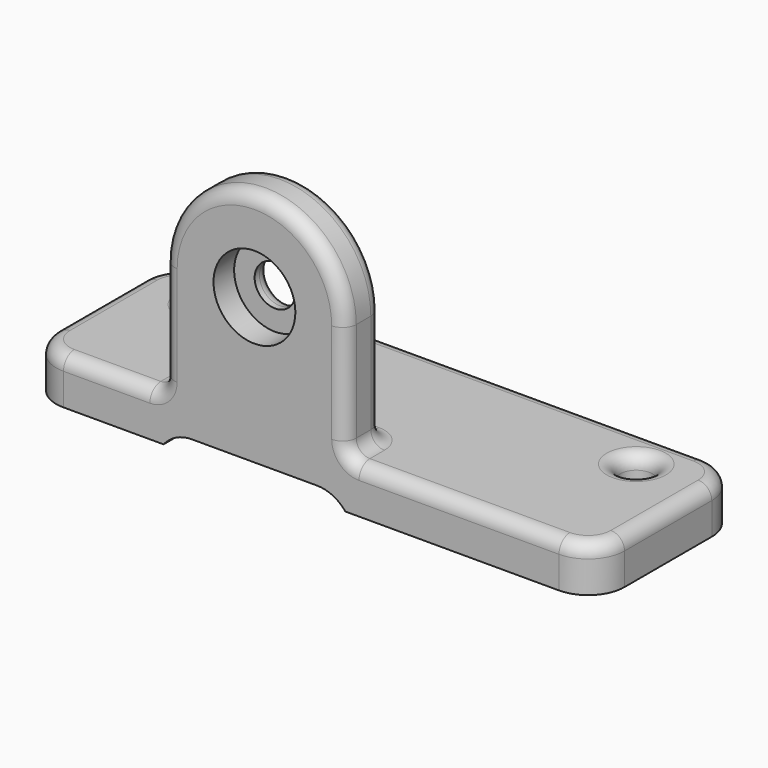
from build123d import *

# Parameters (mm, degrees)
F0_W           = 125
F0_H           = 40
F1_DEPTH       = 10
F3_DEPTH       = 10
F5_D           = 9
F5_CBORE_D     = 18.01
F5_CBORE_DEPTH = 5.68
F6_W           = 40
F6_H           = 3
F7_DEPTH       = 40.001
F8_T1_DEPTH    = 40
F9_R           = 3.2524289183
F10_DEPTH      = 10.001
F11_R          = 3.5
F12_DEPTH      = 25
F13_R          = 8
F14_R          = 3


# Not quite as in the source:
# - a fillet or chamfer that OpenCascade refuses, or shapes differently, is made with other operations: its cross-section is extruded or revolved along the edge and cut away or added


with BuildPart() as f1:
    # F0 (on Top) → F1 (new body)
    with BuildSketch(Plane.XY):
        Rectangle(F0_W, F0_H)
    extrude(amount=F1_DEPTH)

    # F2 (on face) → F3 (join)
    with BuildSketch(Plane.XZ.offset(20)):
        with BuildLine():
            Line((-32.5, 35), (-32.5, 10))
            Line((-32.5, 10), (7.5, 10))
            Line((7.5, 10), (7.5, 35))
            ThreePointArc((7.5, 35), (-12.5, 55), (-32.5, 35))
        make_face()
    extrude(amount=-F3_DEPTH)

    # F5 (through all)
    with Locations(Plane.XZ.offset(20)):
        with Locations((-12.5, 35)):
            CounterBoreHole(F5_D / 2, F5_CBORE_D / 2, F5_CBORE_DEPTH)

    # F6 (on face) → F7 (cut, through all)
    with BuildSketch(Plane.XZ.offset(20)):
        with Locations((-12.5, 1.5)):
            Rectangle(F6_W, F6_H)
    extrude(amount=-F7_DEPTH, mode=Mode.SUBTRACT)

    # F8: fillet of radius 8 on 2 edges, made by hand

    # F8_s2 → F8_t1 (join)
    with BuildSketch(Plane.XZ.offset(-20)):
        with BuildLine():
            ThreePointArc((-32.5, 0), (-29.7191036167, 2.2111025509), (-26.2550020016, 3))
            Line((-26.2550020016, 3), (-32.5, 3))
            Line((-32.5, 3), (-32.5, 0))
        make_face()
        with BuildLine():
            ThreePointArc((1.2550020016, 3), (4.7191036167, 2.2111025509), (7.5, 0))
            Line((7.5, 0), (7.5, 3))
            Line((7.5, 3), (1.2550020016, 3))
        make_face()
    extrude(amount=F8_T1_DEPTH)

    # F9 (on face) → F10 (cut, through all)
    with BuildSketch(Plane.XY.offset(10)):
        with Locations((-47.5, 10)):
            Circle(F9_R)
    extrude(amount=-F10_DEPTH, mode=Mode.SUBTRACT)

    # F11 (on face) → F12 (cut)
    with BuildSketch(Plane.XY.offset(10)):
        with Locations((47.5, 10)):
            Circle(F11_R)
    extrude(amount=-F12_DEPTH, mode=Mode.SUBTRACT)

    # F13
    f13_edges = [f1.edges().sort_by_distance(p)[0] for p in [
        (62.5, -20, 5),
        (-62.5, -20, 5),
        (-62.5, 20, 5),
        (62.5, 20, 5),
    ]]
    fillet(f13_edges, radius=F13_R)

    # F14
    f14_edges = [f1.edges().sort_by_distance(p)[0] for p in [
        (7.5, -15, 10),
        (-32.5, -15, 10),
        (-62.5, 0, 10),
        (-60.156854, 17.656854, 10),
        (-60.156854, -17.656854, 10),
        (0, 20, 10),
        (-43.5, -20, 10),
        (60.156854, 17.656854, 10),
        (62.5, 0, 10),
        (-12.5, -10, 10),
        (60.156854, -17.656854, 10),
        (31, -20, 10),
        (-50.752429, 10, 10),
        (44, 10, 10),
        (-12.5, -10, 55),
        (7.5, -10, 22.5),
        (-32.5, -10, 22.5),
        (-17, -10, 35),
        (-32.5, -20, 22.5),
        (-12.5, -20, 55),
        (7.5, -20, 22.5),
    ]]
    fillet(f14_edges, radius=F14_R)


solid = f1.part
